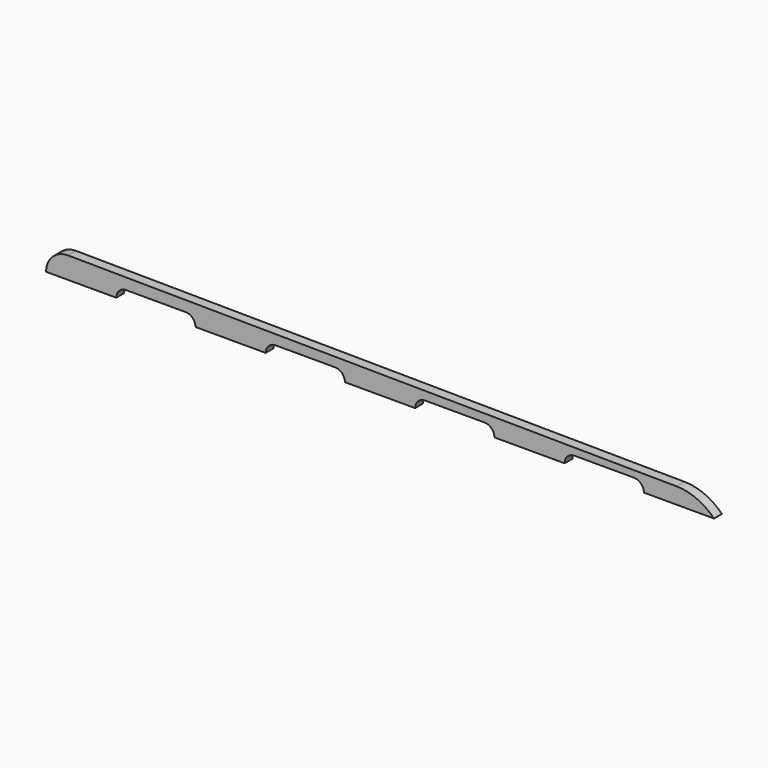
from build123d import *

# Parameters (mm, degrees)
F1_DEPTH = 25
F2_R     = 24.99999
F3_R     = 24.99999
F4_R     = 24.99999
F5_R     = 24.99999


# Not quite as in the source:
# - a fillet or chamfer is up to 0.001 mm smaller than in the source, because OpenCascade refuses the exact size


with BuildPart() as f1:
    # F0 (on Front) → F1 (new body)
    with BuildSketch(Plane.XZ):
        with BuildLine():
            ThreePointArc((55.4895948443, 54.5060273456), (16.4576480368, 38.7445048189), (0.0021987788, 0))
            Line((0.0021987788, 0), (177, 0))
            Line((177, 0), (177, 25))
            Line((177, 25), (377, 25))
            Line((377, 25), (377, 0))
            Line((377, 0), (554, 0))
            Line((554, 0), (554, 25))
            Line((554, 25), (754, 25))
            Line((754, 25), (754, 0))
            Line((754, 0), (931, 0))
            Line((931, 0), (931, 25))
            Line((931, 25), (1131, 25))
            Line((1131, 25), (1131, 0))
            Line((1131, 0), (1308, 0))
            Line((1308, 0), (1308, 25))
            Line((1308, 25), (1508, 25))
            Line((1508, 25), (1508, 0))
            Line((1508, 0), (1685, 0))
            ThreePointArc((1685, 0), (1642.0718401331, 29.7373237733), (1591.0429702736, 40.8364127275))
            Line((1591.0429702736, 40.8364127275), (55.4895948443, 54.5060273456))
        make_face()
    extrude(amount=F1_DEPTH)

    # F2 (radius 25 in the source; OpenCascade refuses exactly that, so slightly less here)
    f2_edges = [f1.edges().sort_by_distance(p)[0] for p in [
        (177, -12.5, 25),
    ]]
    fillet(f2_edges, radius=F2_R)

    # F3 (radius 25 in the source; OpenCascade refuses exactly that, so slightly less here)
    f3_edges = [f1.edges().sort_by_distance(p)[0] for p in [
        (377, -12.5, 25),
    ]]
    fillet(f3_edges, radius=F3_R)

    # F4 (radius 25 in the source; OpenCascade refuses exactly that, so slightly less here)
    f4_edges = [f1.edges().sort_by_distance(p)[0] for p in [
        (754, -12.5, 25),
        (1131, -12.5, 25),
    ]]
    fillet(f4_edges, radius=F4_R)

    # F5 (radius 25 in the source; OpenCascade refuses exactly that, so slightly less here)
    f5_edges = [f1.edges().sort_by_distance(p)[0] for p in [
        (1508, -12.5, 25),
        (554, -12.5, 25),
        (931, -12.5, 25),
        (1308, -12.5, 25),
    ]]
    fillet(f5_edges, radius=F5_R)


solid = f1.part
